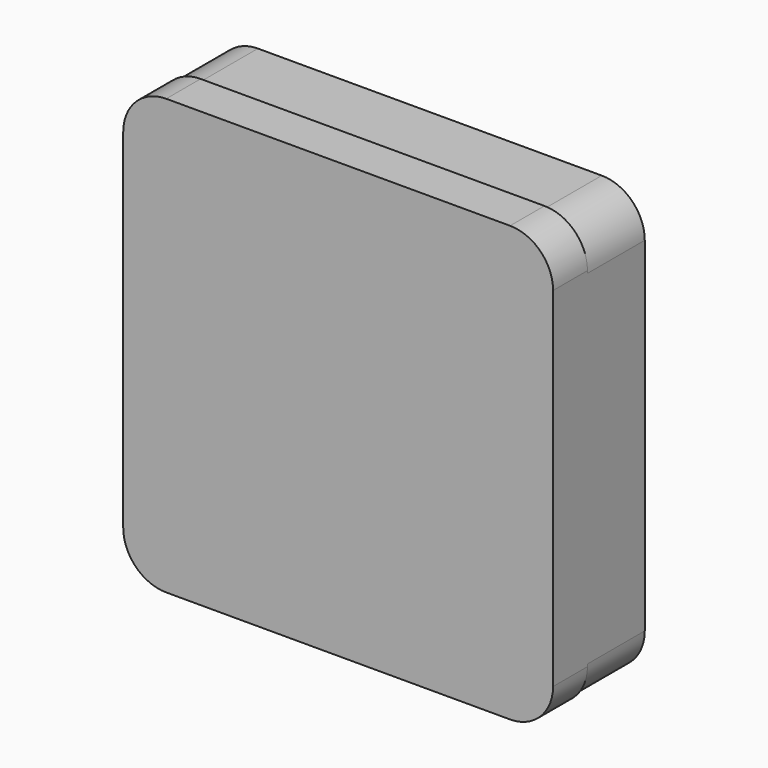
from build123d import *

# Parameters (mm, degrees)
F1_DEPTH = 12.7
F3_D     = 12.3444
F4_R     = 7.62
F5_W     = 76.2
F5_H     = 77.0487710834
F6_DEPTH = 7.62
F7_R     = 7.62


# Not quite as in the source:
# - a feature names something its author has since deleted; it is built from what else it names


with BuildPart() as f1:
    # F0 (on Front) → F1 (new body)
    with BuildSketch(Plane.XZ):
        Polygon((-38.1, -38.1), (38.1, -38.1), (38.1, -30.48), (38.1, 38.1), (-38.1, 38.1), align=None)
    extrude(amount=F1_DEPTH)

    # F3 (through all)
    with Locations(Plane.XZ.offset(12.7)):
        with Locations((-29.1592, 29.1592), (-14.5796, 29.1592), (0, 29.1592), (14.5796, 29.1592), (29.1592, 29.1592), (29.1592, 14.5796), (29.1592, 0), (29.1592, -14.5796), (29.1592, -29.1592), (14.5796, -29.1592), (14.5796, -14.5796), (14.5796, 0), (14.5796, 14.5796), (0, 14.5796), (0, 0), (0, -14.5796), (0, -29.1592), (-14.5796, -29.1592), (-14.5796, -14.5796), (-14.5796, 0), (-14.5796, 14.5796), (-29.1592, 14.5796), (-29.1592, 0), (-29.1592, -14.5796), (-29.1592, -29.1592)):
            Hole(F3_D / 2)

    # F4
    f4_edges = [f1.edges().sort_by_distance(p)[0] for p in [
        (-38.1, -6.35, 38.1),
        (38.1, -6.35, 38.1),
        (38.1, -6.35, -38.1),
        (-38.1, -6.35, -38.1),
    ]]
    fillet(f4_edges, radius=F4_R)

    # F5 (on face) → F6 (join)
    with BuildSketch(Plane.XZ.offset(12.7)):
        Rectangle(F5_W, F5_H)
    extrude(amount=F6_DEPTH)

    # F7
    f7_edges = [f1.edges().sort_by_distance(p)[0] for p in [
        (-38.1, -16.51, 38.524386),
        (38.1, -16.51, 38.524386),
        (38.1, -16.51, -38.524386),
        (-38.1, -16.51, -38.524386),
    ]]
    fillet(f7_edges, radius=F7_R)


solid = f1.part
